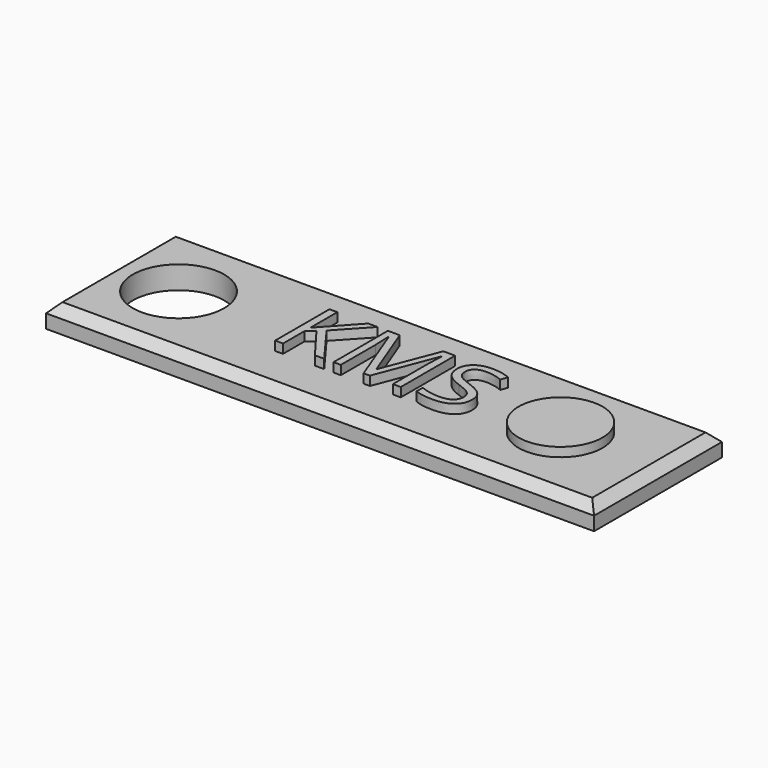
from build123d import *

# Parameters (mm, degrees)
F0_W         = 120
F0_H         = 35
F0_R         = 10
F1_DEPTH     = 5
F2_SIZE      = 2
F4_TEXT_SIZE = 20.8333333333
F6_DEPTH     = 2
F5_R         = 9.1884111706
F7_DEPTH     = 2


# Not quite as in the source:
# - a feature of the source that left no trace in its solid (it failed there, or was rolled back) is left out
# - Text() gives the source's letters only with a copy of the font that has no kerning and outlines rounded to 1/6400 em; it was checked with that copy


with BuildPart() as f1:
    # F0 (on Top) → F1 (new body)
    with BuildSketch(Plane.XY):
        Rectangle(F0_W, F0_H)
        with Locations((-45, 0)):
            Circle(F0_R, mode=Mode.SUBTRACT)
    extrude(amount=F1_DEPTH)

    # F2
    f2_edges = [f1.edges().sort_by_distance(p)[0] for p in [
        (60, 0, 5),
        (0, -17.5, 5),
        (-60, 0, 5),
        (0, 17.5, 5),
    ]]
    chamfer(f2_edges, length=F2_SIZE)

    # F4 (on face) → F6 (join)
    with BuildSketch(Plane.XY.offset(5)):
        with Locations((-20.3460520052, -6.9254449457)):
            Text('KMS', F4_TEXT_SIZE, font='Open Sans', text_align=(TextAlign.LEFT, TextAlign.BOTTOM))
    extrude(amount=F6_DEPTH)

    # F5 (on face) → F7 (join)
    with BuildSketch(Plane.XY.offset(5)):
        with Locations((38.6667773128, 0)):
            Circle(F5_R)
    extrude(amount=F7_DEPTH)


solid = f1.part
